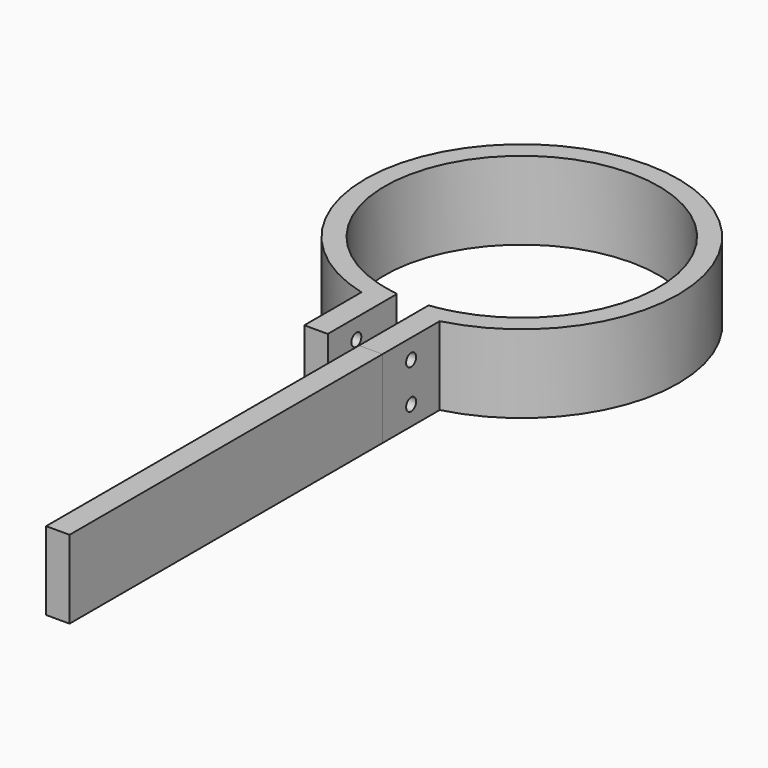
from build123d import *
from build123d import SkipClean  # not in build123d's __all__

# Parameters (mm, degrees)
F1_DEPTH       = 20
F3_D           = 3.2
F3_CBORE_D     = 6
F3_CBORE_DEPTH = 2
F4_W           = 100
F4_H           = 20
F5_DEPTH       = 6


with BuildPart() as f1:
    # F0 (on Top) → F1 (new body)
    with BuildSketch(Plane.XY):
        with BuildLine():
            ThreePointArc((-10, 16.4589803375), (0, 85), (10, 16.4589803375))
            Line((10, 16.4589803375), (10, 11.2701665379))
            ThreePointArc((10, 11.2701665379), (0, 90), (-10, 11.2701665379))
            Line((-10, 11.2701665379), (-10, 16.4589803375))
        make_face()
        with BuildLine():
            ThreePointArc((-4.1759576062, 15.2500161429), (-7.1137080428, 15.7305506627), (-10, 16.4589803375))
            Line((-10, 16.4589803375), (-10, 11.2701665379))
            Line((-10, 11.2701665379), (-10, -7.0000002161))
            Line((-10, -7.0000002161), (-4.00000019, -7.0000002161))
            Line((-4.00000019, -7.0000002161), (-4.00000019, 15))
            Line((-4.00000019, 15), (-4.1759576062, 15.2500161429))
        make_face()
        with BuildLine():
            Line((10, 11.2701665379), (10, 16.4589803375))
            ThreePointArc((10, 16.4589803375), (6.990271983, 15.7051593151), (3.925610649, 15.2208455964))
            Line((3.925610649, 15.2208455964), (4.00000019, 15))
            Line((4.00000019, 15), (4.00000019, -7.0000002161))
            Line((4.00000019, -7.0000002161), (10, -7.0000002161))
            Line((10, -7.0000002161), (10, 11.2701665379))
        make_face()
    extrude(amount=F1_DEPTH)

    # F3 (through all)
    with Locations(Plane(origin=(-10, 0, 0), x_dir=(0, -1, 0), z_dir=(-1, 0, 0))):
        with Locations((-2.1350831609, 5), (-2.1350831609, 15)):
            CounterBoreHole(F3_D / 2, F3_CBORE_D / 2, F3_CBORE_DEPTH)

    # F4 (on face) → F5 (join)
    with BuildSketch(Plane.YZ.offset(10)):
        with Locations((-57.0000002161, 10)):
            Rectangle(F4_W, F4_H)
    with SkipClean():  # cleaning this boolean's faces spoils the solid; the shape is the same uncleaned
        extrude(amount=-F5_DEPTH)


solid = f1.part
